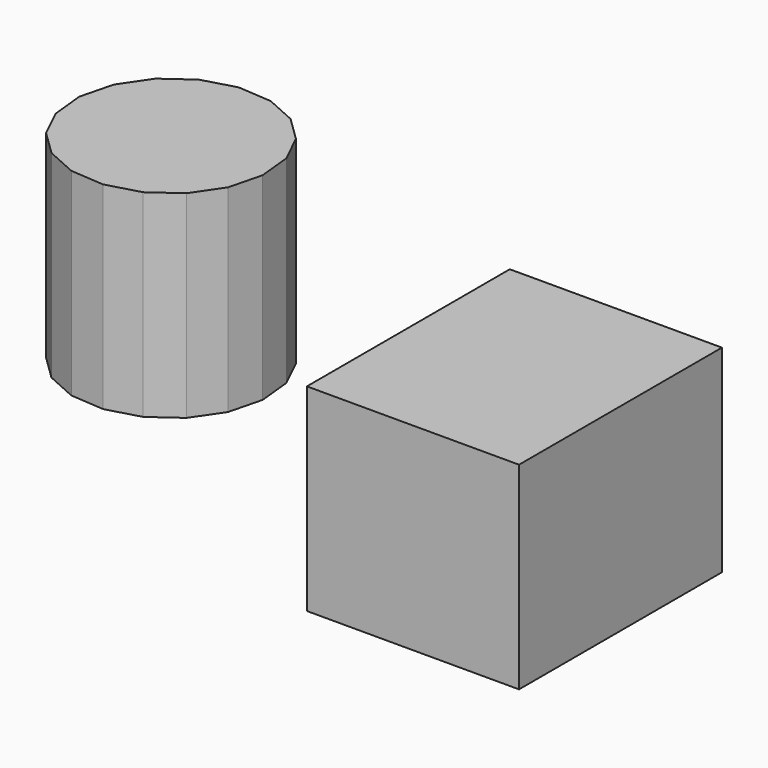
from build123d import *

# Parameters (mm, degrees)
F1_DEPTH = 25.4
F2_DEPTH = 25.4
F3_W     = 54.4781722128
F3_H     = 65.1334398426
F4_DEPTH = 25.4
F6_DEPTH = 25.4


# Not quite as in the source:
# - a feature of the source that left no trace in its solid (it failed there, or was rolled back) is left out


with BuildPart() as f1:
    # F0 (on Top) → F1 (new body)
    with BuildSketch(Plane.XY):
        Polygon((-34.6092643811, 30.9926864128), (-38.4029460476, 38.8350266595), (-44.6500790503, 44.9069003716), (-52.5971669514, 48.4759499683), (-61.2856736633, 49.1116953946), (-69.667637048, 46.7374563695), (-76.7320686166, 41.6396011594), (-81.6268936621, 34.4330063391), (-83.7617240441, 25.9868936018), (-82.8790677116, 17.319988795), (-79.0853860452, 9.4776485484), (-72.8382530424, 3.4057748362), (-64.8911651414, -0.1632747605), (-56.2026584294, -0.7990201868), (-47.8206950447, 1.5752188384), (-40.7562634761, 6.6730740484), (-35.8614384306, 13.8796688688), (-33.7266080487, 22.3257816061), align=None)
    extrude(amount=F1_DEPTH)

    # F2 (add): a face of the model
    f2_faces = [f1.faces().sort_by_distance(p)[0] for p in [
        (-58.7441660464, 24.1563376039, 25.4),
    ]]
    extrude(f2_faces, amount=F2_DEPTH)


with BuildPart() as f4:
    # F3 (on Top) → F4 (new body)
    with BuildSketch(Plane.XY):
        with Locations((27.2390861064, 26.9183467608)):
            Rectangle(F3_W, F3_H)
    extrude(amount=F4_DEPTH)

    # F6 (add): a face of the model
    f6_faces = [f4.faces().sort_by_distance(p)[0] for p in [
        (27.2390861064, 26.9183467608, 0),
    ]]
    extrude(f6_faces, amount=F6_DEPTH)


solid = Compound([f1.part, f4.part])
